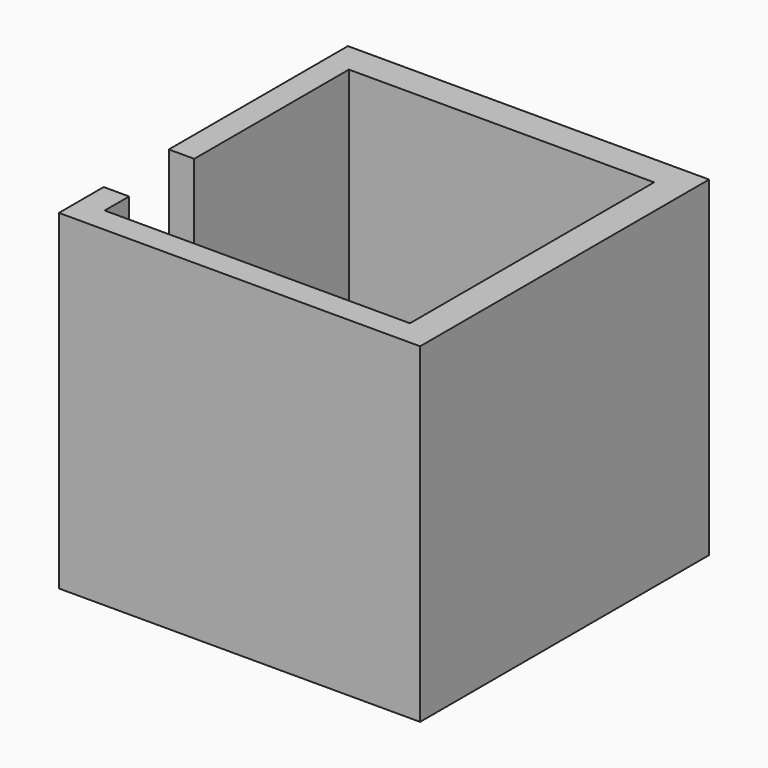
from build123d import *

# Parameters (mm, degrees)
F1_DEPTH = 3000
F2_W     = 3550
F2_H     = 3550
F3_DEPTH = 250


# Not quite as in the source:
# - a feature names something its author has since deleted; it is built from what else it names


with BuildPart() as f1:
    # F0 (on Top) → F1 (new body)
    with BuildSketch(Plane.XY):
        Polygon((3000, 0), (0, 0), (0, 300), (-250, 300), (-250, -250), (3300, -250), (3300, 3300), (-250, 3300), (-250, 1100), (0, 1100), (0, 3000), (3000, 3000), align=None)
    extrude(amount=F1_DEPTH)

    # F2 (on Top) → F3 (join)
    with BuildSketch(Plane.XY):
        with Locations((1525, 1525)):
            Rectangle(F2_W, F2_H)
    extrude(amount=-F3_DEPTH)


solid = f1.part
